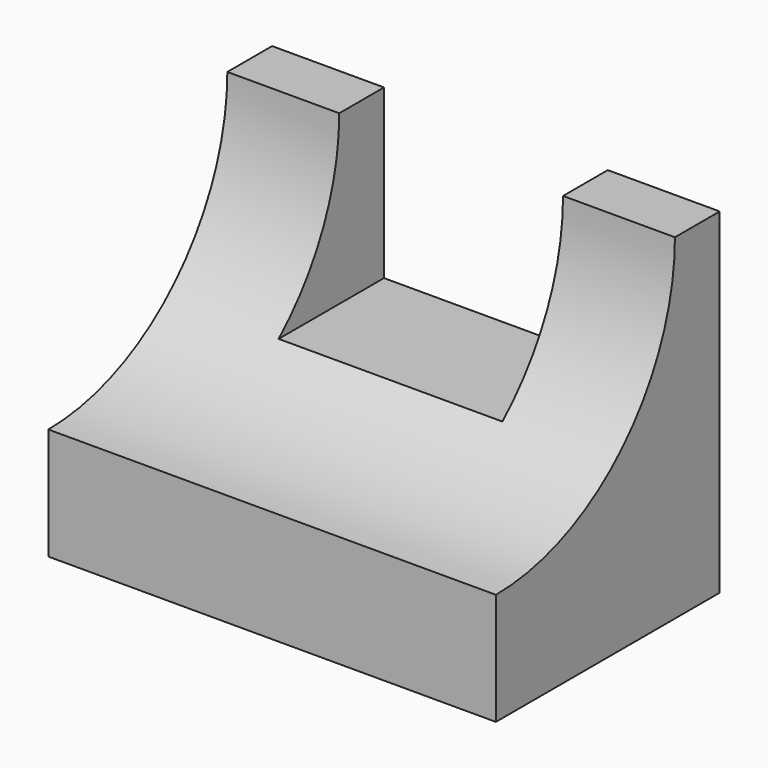
from build123d import *

# Parameters (mm, degrees)
F0_W     = 31.75
F0_H     = 38.1
F1_DEPTH = 50.8
F3_DEPTH = 50.801
F4_W     = 25.4
F4_H     = 19.05
F5_DEPTH = 31.751


# Not quite as in the source:
# - a feature names something its author has since deleted; it is built from what else it names


with BuildPart() as f1:
    # F0 (on Right) → F1 (new body)
    with BuildSketch(Plane.YZ):
        with Locations((15.875, 19.05)):
            Rectangle(F0_W, F0_H)
    extrude(amount=F1_DEPTH)

    # F2 (on face) → F3 (cut, through all)
    with BuildSketch(Plane.YZ.offset(50.8)):
        with BuildLine():
            Line((0, 38.1), (25.4, 38.1))
            ThreePointArc((25.4, 38.1), (-17.9605122421, 56.0605122421), (0, 12.7))
            Line((0, 12.7), (0, 38.1))
        make_face()
        with BuildLine():
            ThreePointArc((0, 12.7), (17.9605122421, 20.1394877579), (25.4, 38.1))
            Line((25.4, 38.1), (0, 38.1))
            Line((0, 38.1), (0, 12.7))
        make_face()
    extrude(amount=-F3_DEPTH, mode=Mode.SUBTRACT)

    # F4 (on face) → F5 (cut, through all)
    with BuildSketch(Plane(origin=(0, 31.75, 0), x_dir=(-1, 0, 0), z_dir=(0, 1, 0))):
        with Locations((-25.4, 28.575)):
            Rectangle(F4_W, F4_H)
    extrude(amount=-F5_DEPTH, mode=Mode.SUBTRACT)


solid = f1.part
